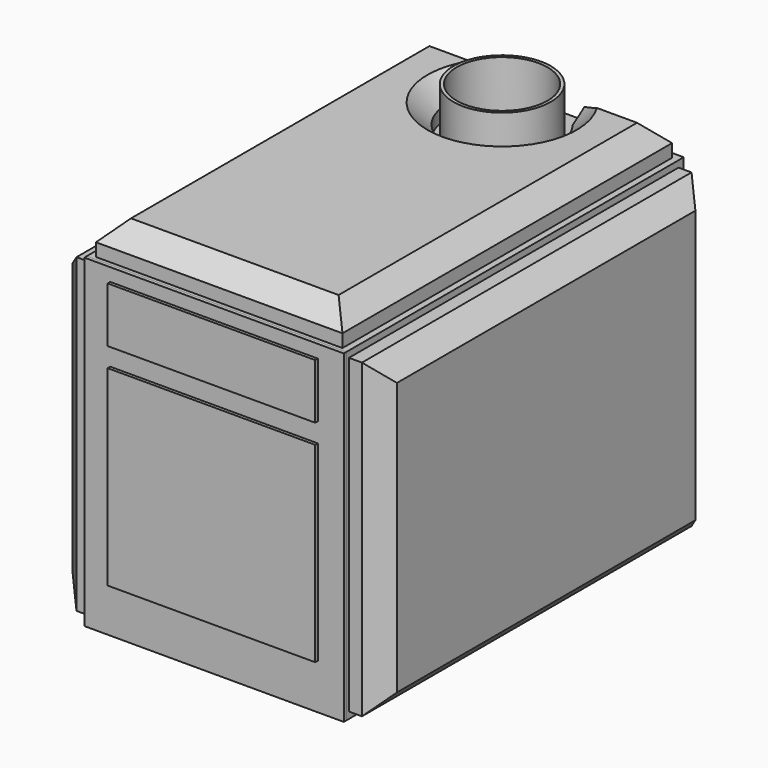
from build123d import *

# Parameters (mm, degrees)
F1_W          = 400
F1_H          = 650
F2_DEPTH      = 500
F3_T          = -5
F4_W          = 390
F4_H          = 5
F5_DEPTH      = 600
F6_W          = 390
F6_H          = 5
F7_DEPTH      = 600
F9_DEPTH      = 645
F10_R         = 75
F11_DEPTH     = 75
F12_R         = 70
F13_DEPTH     = 80
F14_W         = 400
F14_H         = 500
F14_W_2       = 300
F14_H_2       = 275
F14_H_3       = 65
F15_DEPTH     = 5
F16_W         = 320
F16_H         = 85
F17_DEPTH     = 5
F16_H_2       = 295
F18_W         = 635
F18_H         = 480
F19_DEPTH     = 50
F22_DEPTH     = 50
F23_C1_SIZE   = 30
F23_C2_SIZE   = 30
F23_C3_SIZE   = 30
F23_C4_SIZE   = 30
F23_2_C1_SIZE = 30
F23_2_C2_SIZE = 30
F23_2_C3_SIZE = 30
F23_2_C4_SIZE = 30
F23_2_C5_SIZE = 30
F23_2_C6_SIZE = 30
F23_3_C1_SIZE = 30
F23_3_C2_SIZE = 30
F23_3_C3_SIZE = 30
F23_3_C4_SIZE = 30


with BuildPart() as f2:
    # F1 (on Top) → F2 (new body)
    with BuildSketch(Plane.XY):
        with Locations((0, 325)):
            Rectangle(F1_W, F1_H)
    extrude(amount=F2_DEPTH)

    # F3
    f3_openings = [f2.faces().sort_by_distance(p)[0] for p in [
        (0, 0, 250),
    ]]
    offset(amount=F3_T, openings=f3_openings)

    # F10 (on face) → F11 (join)
    with BuildSketch(Plane.XY.offset(500)):
        with Locations((0, 550)):
            Circle(F10_R)
    extrude(amount=F11_DEPTH)

    # F12 (on face) → F13 (cut, through all)
    with BuildSketch(Plane.XY.offset(575)):
        with Locations((0, 550)):
            Circle(F12_R)
    extrude(amount=-F13_DEPTH, mode=Mode.SUBTRACT)


with BuildPart() as f5:
    # F4 (on face) → F5 (new body)
    with BuildSketch(Plane.XZ.offset(-645)):
        with Locations((0, 442.5)):
            Rectangle(F4_W, F4_H)
    extrude(amount=F5_DEPTH)


with BuildPart() as f7:
    # F6 (on face) → F7 (new body)
    with BuildSketch(Plane.XZ):
        with Locations((0, 387.5)):
            Rectangle(F6_W, F6_H)
    extrude(amount=-F7_DEPTH)


with BuildPart() as f9:
    # F8 (on face) → F9 (new body, through all)
    with BuildSketch(Plane.XZ.offset(-645)):
        Polygon((-170, 52), (-170, 55), (-195, 55), (-195, 30), (-192, 30), (-192, 52), align=None)
    extrude(amount=F9_DEPTH)


with BuildPart() as f9b:
    # F8 (on face) → F9, piece 2 (new body, through all)
    with BuildSketch(Plane.XZ.offset(-645)):
        Polygon((192, 30), (195, 30), (195, 55), (170, 55), (170, 52), (192, 52), align=None)
    extrude(amount=F9_DEPTH)


with BuildPart() as f15:
    # F14 (on face) → F15 (new body)
    with BuildSketch(Plane.XZ):
        with Locations((0, 250)):
            Rectangle(F14_W, F14_H)
        with Locations((0, 217.5)):
            Rectangle(F14_W_2, F14_H_2, mode=Mode.SUBTRACT)
        with Locations((0, 437.5)):
            Rectangle(F14_W_2, F14_H_3, mode=Mode.SUBTRACT)
    extrude(amount=F15_DEPTH)


with BuildPart() as f17:
    # F16 (on face) → F17 (new body)
    with BuildSketch(Plane.XZ.offset(5)):
        with Locations((0, 437.5)):
            Rectangle(F16_W, F16_H)
    extrude(amount=F17_DEPTH)


with BuildPart() as f17b:
    # F16 (on face) → F17, piece 2 (new body)
    with BuildSketch(Plane.XZ.offset(5)):
        with Locations((0, 217.5)):
            Rectangle(F16_W, F16_H_2)
    extrude(amount=F17_DEPTH)


with BuildPart() as f19:
    # F18 (on face) → F19 (new body)
    with BuildSketch(Plane(origin=(-200, 0, 0), x_dir=(0, -1, 0), z_dir=(-1, 0, 0))):
        with Locations((-322.5, 250)):
            Rectangle(F18_W, F18_H)
    extrude(amount=F19_DEPTH)


with BuildPart() as f20_1:
    # F20: instance of F19
    add(f19.part.mirror(Plane.YZ))

    # F23#3: chamfer of 30 on 4 edges, made by hand

    # F23_3_c1
    f23_3_c1_edges = [f20_1.edges().sort_by_distance(p)[0] for p in [
        (250, 322.5, 490),
    ]]
    chamfer(f23_3_c1_edges, length=F23_3_C1_SIZE)

    # F23_3_c2
    f23_3_c2_edges = [f20_1.edges().sort_by_distance(p)[0] for p in [
        (250, 640, 235),
    ]]
    chamfer(f23_3_c2_edges, length=F23_3_C2_SIZE)

    # F23_3_c3
    f23_3_c3_edges = [f20_1.edges().sort_by_distance(p)[0] for p in [
        (250, 307.5, 10),
    ]]
    chamfer(f23_3_c3_edges, length=F23_3_C3_SIZE)

    # F23_3_c4
    f23_3_c4_edges = [f20_1.edges().sort_by_distance(p)[0] for p in [
        (250, 5, 250),
    ]]
    chamfer(f23_3_c4_edges, length=F23_3_C4_SIZE)


with BuildPart() as f22:
    # F21 (on face) → F22 (new body)
    with BuildSketch(Plane.XY.offset(500)):
        with BuildLine():
            Line((-67.0872659549, 640), (-190, 640))
            Line((-190, 640), (-190, 5))
            Line((-190, 5), (190, 5))
            Line((190, 5), (190, 640))
            Line((190, 640), (67.0872659549, 640))
            Line((67.0872659549, 640), (67.0872659549, 602.1948153239))
            ThreePointArc((67.0872659549, 602.1948153239), (0, 465), (-67.0872659549, 602.1948153239))
            Line((-67.0872659549, 602.1948153239), (-67.0872659549, 640))
        make_face()
    extrude(amount=F22_DEPTH)

    # F23#2: chamfer of 30 on 8 edges, made by hand

    # F23_2_c1
    f23_2_c1_edges = [f22.edges().sort_by_distance(p)[0] for p in [
        (-128.5436329775, 640, 550),
    ]]
    chamfer(f23_2_c1_edges, length=F23_2_C1_SIZE)

    # F23_2_c2
    f23_2_c2_edges = [f22.edges().sort_by_distance(p)[0] for p in [
        (-190, 307.5, 550),
    ]]
    chamfer(f23_2_c2_edges, length=F23_2_C2_SIZE)

    # F23_2_c3
    f23_2_c3_edges = [f22.edges().sort_by_distance(p)[0] for p in [
        (15, 5, 550),
    ]]
    chamfer(f23_2_c3_edges, length=F23_2_C3_SIZE)

    # F23_2_c4
    f23_2_c4_edges = [f22.edges().sort_by_distance(p)[0] for p in [
        (190, 337.5, 550),
    ]]
    chamfer(f23_2_c4_edges, length=F23_2_C4_SIZE)

    # F23_2_c5
    f23_2_c5_edges = [f22.edges().sort_by_distance(p)[0] for p in [
        (113.5436329775, 640, 550),
    ]]
    chamfer(f23_2_c5_edges, length=F23_2_C5_SIZE)

    # F23_2_c6
    f23_2_c6_edges = [f22.edges().sort_by_distance(p)[0] for p in [
        (0, 465, 550),
    ]]
    chamfer(f23_2_c6_edges, length=F23_2_C6_SIZE)


with BuildPart() as f19_1:
    add(f19.part)

    # F23: chamfer of 30 on 4 edges, made by hand

    # F23_c1
    f23_c1_edges = [f19_1.edges().sort_by_distance(p)[0] for p in [
        (-250, 322.5, 490),
    ]]
    chamfer(f23_c1_edges, length=F23_C1_SIZE)

    # F23_c2
    f23_c2_edges = [f19_1.edges().sort_by_distance(p)[0] for p in [
        (-250, 640, 235),
    ]]
    chamfer(f23_c2_edges, length=F23_C2_SIZE)

    # F23_c3
    f23_c3_edges = [f19_1.edges().sort_by_distance(p)[0] for p in [
        (-250, 307.5, 10),
    ]]
    chamfer(f23_c3_edges, length=F23_C3_SIZE)

    # F23_c4
    f23_c4_edges = [f19_1.edges().sort_by_distance(p)[0] for p in [
        (-250, 5, 250),
    ]]
    chamfer(f23_c4_edges, length=F23_C4_SIZE)


solid = Compound([f2.part, f5.part, f7.part, f9.part, f9b.part, f15.part, f17.part, f17b.part, f20_1.part, f22.part, f19_1.part])
